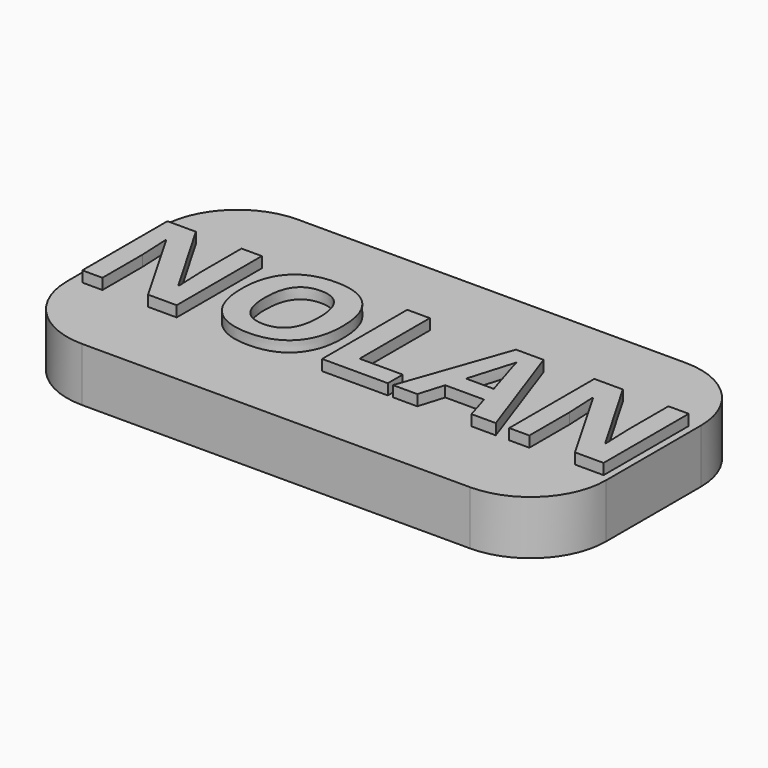
from build123d import *

# Parameters (mm, degrees)
F0_W         = 50
F0_H         = 25
F1_DEPTH     = 5
F2_TEXT_SIZE = 13.831264434
F3_DEPTH     = 1
F4_R         = 7


# Not quite as in the source:
# - Text() gives the source's letters only with a copy of the font that has no kerning and outlines rounded to 1/6400 em; it was checked with that copy


with BuildPart() as f1:
    # F0 (on Top) → F1 (new body)
    with BuildSketch(Plane.XY):
        with Locations((25, 12.5)):
            Rectangle(F0_W, F0_H)
    extrude(amount=F1_DEPTH)

    # F2 (on face) → F3 (join)
    with BuildSketch(Plane.XY.offset(5)):
        with Locations((-0.2550244024, 7.5207448038)):
            Text('NOLAN', F2_TEXT_SIZE, font='Open Sans', font_style=FontStyle.BOLD, text_align=(TextAlign.LEFT, TextAlign.BOTTOM))
    extrude(amount=F3_DEPTH)

    # F4
    f4_edges = [f1.edges().sort_by_distance(p)[0] for p in [
        (0, 25, 2.5),
        (0, 0, 2.5),
        (50, 25, 2.5),
        (50, 0, 2.5),
    ]]
    fillet(f4_edges, radius=F4_R)


solid = f1.part
